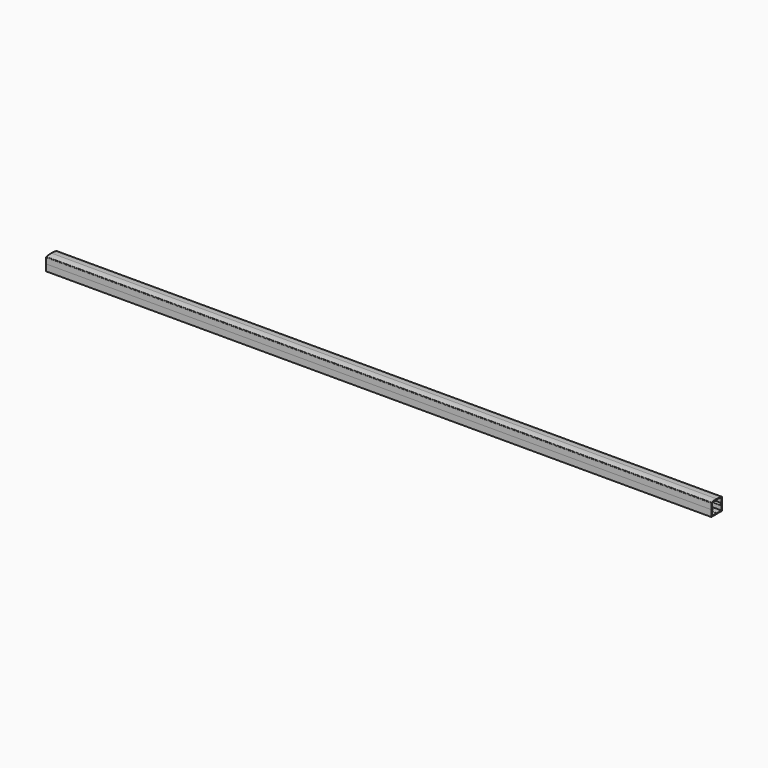
from build123d import *

# Parameters (mm, degrees)
F2_DEPTH = 1000
F4_DEPTH = 1000


with BuildPart() as f2:
    # F1 (on Right) → F2 (new body)
    with BuildSketch(Plane.YZ):
        with BuildLine():
            Line((0.125, -9), (0, -10))
            Line((0, -10), (10, -10))
            Line((10, -10), (10, -0.2))
            Line((10, -0.2), (9, -0.2))
            ThreePointArc((9, -0.2), (8.5, -0.7), (9, -1.2))
            ThreePointArc((9, -1.2), (9.5, -1.7), (9, -2.2))
            Line((9, -2.2), (9, -9))
            Line((9, -9), (0.125, -9))
        make_face()
    extrude(amount=F2_DEPTH)


with BuildPart() as f4:
    # F3 (on Right) → F4 (new body)
    with BuildSketch(Plane.YZ):
        with BuildLine():
            Line((9, -0.2), (10, -0.2))
            Line((10, -0.2), (10, 8.1663783152))
            ThreePointArc((10, 8.1663783152), (9.7693092582, 8.8052548802), (9.1836734694, 9.1493656277))
            ThreePointArc((9.1836734694, 9.1493656277), (4.6114920912, 9.7868872364), (0, 10))
            Line((0, 10), (0, 9))
            ThreePointArc((0, 9), (4.5192622493, 8.7911494917), (9, 8.1663783152))
            Line((9, 8.1663783152), (9, 0.8))
            ThreePointArc((9, 0.8), (7.5, -0.7), (9, -2.2))
            ThreePointArc((9, -2.2), (9.5, -1.7), (9, -1.2))
            ThreePointArc((9, -1.2), (8.5, -0.7), (9, -0.2))
        make_face()
    extrude(amount=F4_DEPTH)

    # F6: F4 across plane


with BuildPart() as f5_1:
    # F5: instance of F2
    add(f2.part.mirror(Plane.XZ))


with BuildPart() as f4_1:
    add(f4.part)
    add(f4.part.mirror(Plane.XZ))


solid = Compound([f2.part, f5_1.part, f4_1.part])
